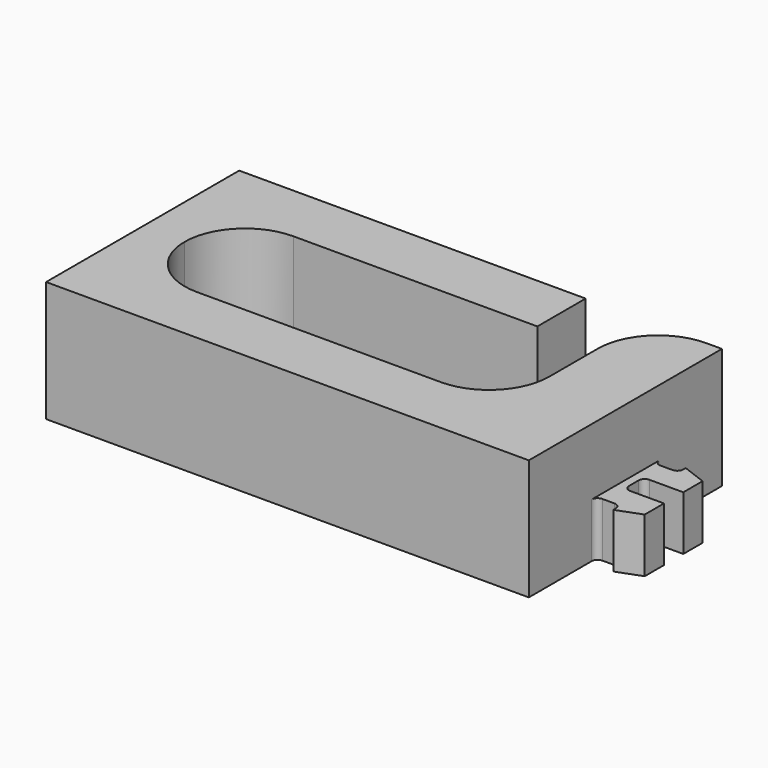
from build123d import *

# Parameters (mm, degrees)
F0_W     = 22.0889396991
F0_H     = 5
F1_DEPTH = 10
F0_W_2   = 2
F0_H_2   = 2
F0_W_3   = 0.7
F2_DEPTH = 4.5
F3_R     = 4.99999
F4_R     = 0.5


# Not quite as in the source:
# - a fillet or chamfer is up to 0.001 mm smaller than in the source, because OpenCascade refuses the exact size


with BuildPart() as f1:
    # F0 (on Top) → F1 (new body)
    with BuildSketch(Plane.XY):
        Polygon((-0.9434188306, 20), (-0.9434188306, 0), (5.6756753474, 0), (5.6756753474, 5), (2.5402316824, 5), (2.5402316824, 15), (5.6756753474, 15), (5.6756753474, 20), align=None)
        Polygon((5.6756753474, 5), (5.6756753474, 0), (39.0565811694, 0), (39.0565811694, 7), (39.0565811694, 9), (39.0565811694, 11), (39.0565811694, 13), (39.0565811694, 20), (32.7646150465, 20), (32.7646150465, 15), (32.7646150465, 5), align=None)
        with Locations((16.720145197, 17.5)):
            Rectangle(F0_W, F0_H)
    extrude(amount=F1_DEPTH)

    # F0 (on Top) → F2 (join)
    with BuildSketch(Plane.XY):
        Polygon((39.0565811694, 9), (39.0565811694, 7), (41.0565811694, 7), (41.0565811694, 9), (39.7565811694, 9), align=None)
        with Locations((42.0565811694, 8)):
            Rectangle(F0_W_2, F0_H_2)
        Polygon((43.0565811694, 7), (41.0565811694, 7), (41.0565811694, 6.25), align=None)
        Polygon((39.0565811694, 13), (39.0565811694, 11), (39.7565811694, 11), (41.0565811694, 11), (41.0565811694, 13), align=None)
        with Locations((42.0565811694, 12)):
            Rectangle(F0_W_2, F0_H_2)
        Polygon((41.0565811694, 13.75), (41.0565811694, 13), (43.0565811694, 13), align=None)
        with Locations((39.4065811694, 10)):
            Rectangle(F0_W_3, F0_H_2)
    extrude(amount=F2_DEPTH)

    # F3 (radius 5 in the source; OpenCascade refuses exactly that, so slightly less here)
    f3_edges = [f1.edges().sort_by_distance(p)[0] for p in [
        (2.540232, 15, 5),
        (2.540232, 5, 5),
        (32.764615, 5, 5),
        (32.764615, 20, 5),
    ]]
    fillet(f3_edges, radius=F3_R)

    # F4
    f4_edges = [f1.edges().sort_by_distance(p)[0] for p in [
        (39.056581, 13, 2.25),
        (39.056581, 7, 2.25),
        (41.056581, 7, 2.25),
        (41.056581, 13, 2.25),
        (39.756581, 11, 2.25),
        (39.756581, 9, 2.25),
    ]]
    fillet(f4_edges, radius=F4_R)


solid = f1.part
